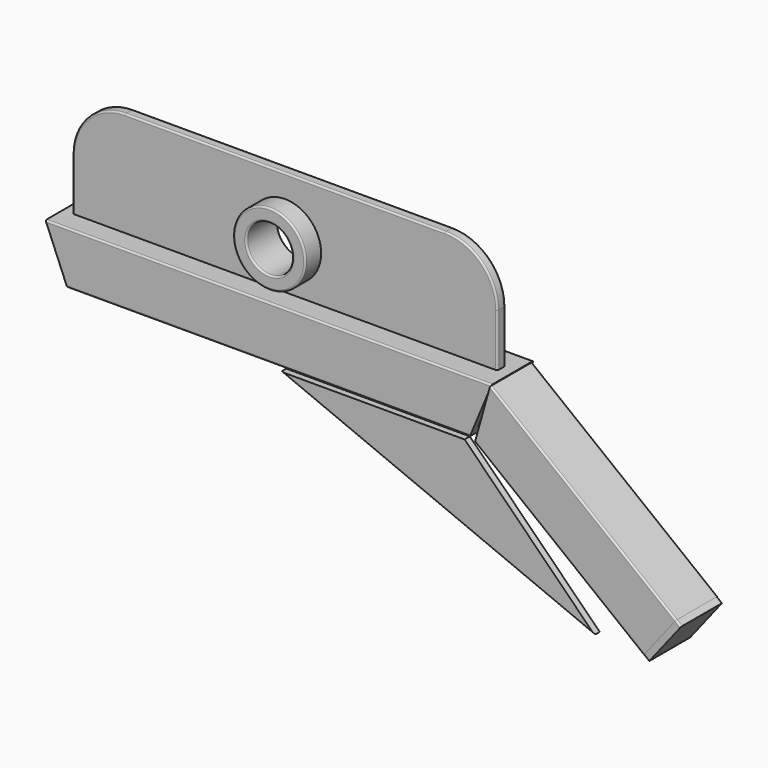
from build123d import *

# Parameters (mm, degrees)
F0_W      = 50.8
F0_H      = 50.8
F0_W_2    = 38.0999986082
F0_H_2    = 38.0999993041
F1_DEPTH  = 215.9
F3_DEPTH  = 50.801
F6_W      = 50.8
F6_H      = 50.8
F6_W_2    = 38.1000041962
F6_H_2    = 38.1000041962
F7_DEPTH  = 228.6
F9_DEPTH  = 50.801
F11_DEPTH = 6.35
F12_W     = 411.099
F12_H     = 9.525
F13_DEPTH = 101.6
F14_R     = 50.8
F15_R     = 22.225
F16_DEPTH = 25.4
F17_R     = 34.925
F17_R_2   = 22.225
F18_DEPTH = 19.05
F20_R     = 1.651
F20_2_R   = 1.651
F20_3_R   = 1.651
F20_4_R   = 1.651
F21_R     = 1.651
F22_W     = 38.1000041962
F22_H     = 38.1000041962
F23_DEPTH = 6.35


with BuildPart() as f1:
    # F0 (on Right) → F1 (new body, symmetric)
    with BuildSketch(Plane.YZ):
        with Locations((-18.0143257603, 3.3626770601)):
            Rectangle(F0_W, F0_H)
        with Locations((-18.0143257603, 3.362677408)):
            Rectangle(F0_W_2, F0_H_2, mode=Mode.SUBTRACT)
    extrude(amount=F1_DEPTH, both=True)

    # F2 (on face) → F3 (cut, through all)
    with BuildSketch(Plane(origin=(0, 7.3856742397, 0), x_dir=(-1, 0, 0), z_dir=(0, 1, 0))):
        Polygon((-194.8579510314, -22.0373229399), (-215.9, 28.7626770601), (-215.9, -22.0373229399), align=None)
        Polygon((215.9, -22.0373229399), (215.9, 28.7626770601), (194.8579510314, -22.0373229399), align=None)
    extrude(amount=-F3_DEPTH, mode=Mode.SUBTRACT)

    # F20
    f20_edges = [f1.edges().sort_by_distance(p)[0] for p in [
        (0, -43.414326, -22.037323),
        (0, -43.414326, 28.762677),
        (0, 7.385674, -22.037323),
        (0, 7.385674, 28.762677),
    ]]
    fillet(f20_edges, radius=F20_R)


with BuildPart() as f7:
    # F6 (on face) → F7 (new body)
    with BuildSketch(Plane(origin=(119.5313421825, 0, -93.9048466977), x_dir=(0, -1, 0), z_dir=(-0.7863587226, 0, 0.6177701509))):
        with Locations((19.0380490385, 129.6261847019)):
            Rectangle(F6_W, F6_H)
        with Locations((19.0380490385, 129.6261847019)):
            Rectangle(F6_W_2, F6_H_2, mode=Mode.SUBTRACT)
    extrude(amount=-F7_DEPTH)

    # F8 (on face) → F9 (cut, through all)
    with BuildSketch(Plane(origin=(0, 6.3619509615, 0), x_dir=(-1, 0, 0), z_dir=(0, 1, 0))):
        Polygon((-183.9191680339, -11.9456772311), (-215.3018916998, 28.0013458784), (-200.4657667823, -24.9448269977), align=None)
    extrude(amount=-F9_DEPTH, mode=Mode.SUBTRACT)

    # F20#2
    f20_2_edges = [f7.edges().sort_by_distance(p)[0] for p in [
        (282.073269, -44.438049, -89.05638),
        (305.182694, -44.438049, -42.609782),
        (305.182694, 6.361951, -42.609782),
        (282.073269, 6.361951, -89.05638),
    ]]
    fillet(f20_2_edges, radius=F20_2_R)


with BuildPart() as f11:
    # F10 (on face) → F11 (new body)
    with BuildSketch(Plane.XZ.offset(43.4143257603)):
        Polygon((320.5815367264, -147.7609086349), (194.8579510314, -22.0373229399), (17.0579510314, -22.0373229399), align=None)
    extrude(amount=F11_DEPTH)

    # F20#3
    f20_3_edges = [f11.edges().sort_by_distance(p)[0] for p in [
        (168.819744, -49.764326, -84.899116),
    ]]
    fillet(f20_3_edges, radius=F20_3_R)


with BuildPart() as f13:
    # F12 (on face) → F13 (new body)
    with BuildSketch(Plane.XY.offset(28.7626770601)):
        with Locations((-0.8255, -17.6774282008)):
            Rectangle(F12_W, F12_H)
    extrude(amount=F13_DEPTH)

    # F14
    f14_edges = [f13.edges().sort_by_distance(p)[0] for p in [
        (-206.375, -17.677428, 130.362677),
        (204.724, -17.677428, 130.362677),
    ]]
    fillet(f14_edges, radius=F14_R)

    # F15 (on face) → F16 (cut)
    with BuildSketch(Plane.XZ.offset(22.4399282008)):
        with Locations((-0.8255, 73.2126770601)):
            Circle(F15_R)
    extrude(amount=-F16_DEPTH, mode=Mode.SUBTRACT)


with BuildPart() as f18:
    # F17 (on face) → F18 (new body, symmetric)
    with BuildSketch(Plane.XZ.offset(22.4399282008)):
        with Locations((-0.8255, 73.2126770601)):
            Circle(F17_R)
        with Locations((-0.8255, 73.2126770601)):
            Circle(F17_R_2, mode=Mode.SUBTRACT)
    extrude(amount=F18_DEPTH, both=True)


with BuildPart() as f13_1:
    add(f13.part)

    # F19: cut F18
    add(f18.part, mode=Mode.SUBTRACT)

    # F20#4
    f20_4_edges = [f13_1.edges().sort_by_distance(p)[0] for p in [
        (204.724, -12.914928, 54.162677),
        (189.845024, -12.914928, 115.483702),
        (204.724, -22.439928, 54.162677),
    ]]
    fillet(f20_4_edges, radius=F20_4_R)


with BuildPart() as f18_1:
    add(f18.part)

    # F21
    f21_edges = [f18_1.edges().sort_by_distance(p)[0] for p in [
        (-23.0505, -3.389928, 73.212677),
        (-35.7505, -3.389928, 73.212677),
        (-23.0505, -41.489928, 73.212677),
        (-35.7505, -41.489928, 73.212677),
    ]]
    fillet(f21_edges, radius=F21_R)


with BuildPart() as f23:
    # F22 (on face) → F23 (new body)
    with BuildSketch(Plane(origin=(299.2929461753, 0, -235.1271031941), x_dir=(0, 1, 0), z_dir=(0.7863587226, 0, -0.6177701509))):
        with BuildLine():
            Line((5.1096215189, 105.1218711495), (5.1096215189, 154.9773278874))
            ThreePointArc((5.1096215189, 154.9773278874), (4.9117775046, 155.0139249802), (4.7109509615, 155.0261847019))
            Line((4.7109509615, 155.0261847019), (-42.7870490385, 155.0261847019))
            ThreePointArc((-42.7870490385, 155.0261847019), (-43.9544823342, 154.5426179977), (-44.4380490385, 153.3751847019))
            Line((-44.4380490385, 153.3751847019), (-44.4380490385, 105.8771847019))
            ThreePointArc((-44.4380490385, 105.8771847019), (-44.3916713568, 105.4886126807), (-44.2551438711, 105.1218711495))
            Line((-44.2551438711, 105.1218711495), (5.1096215189, 105.1218711495))
        make_face()
        with Locations((-19.0380490385, 129.6261847019)):
            Rectangle(F22_W, F22_H, mode=Mode.SUBTRACT)
        with Locations((-19.0380490385, 129.6261847019)):
            Rectangle(F22_W, F22_H)
    extrude(amount=F23_DEPTH)


solid = Compound([f1.part, f7.part, f11.part, f13_1.part, f18_1.part, f23.part])
